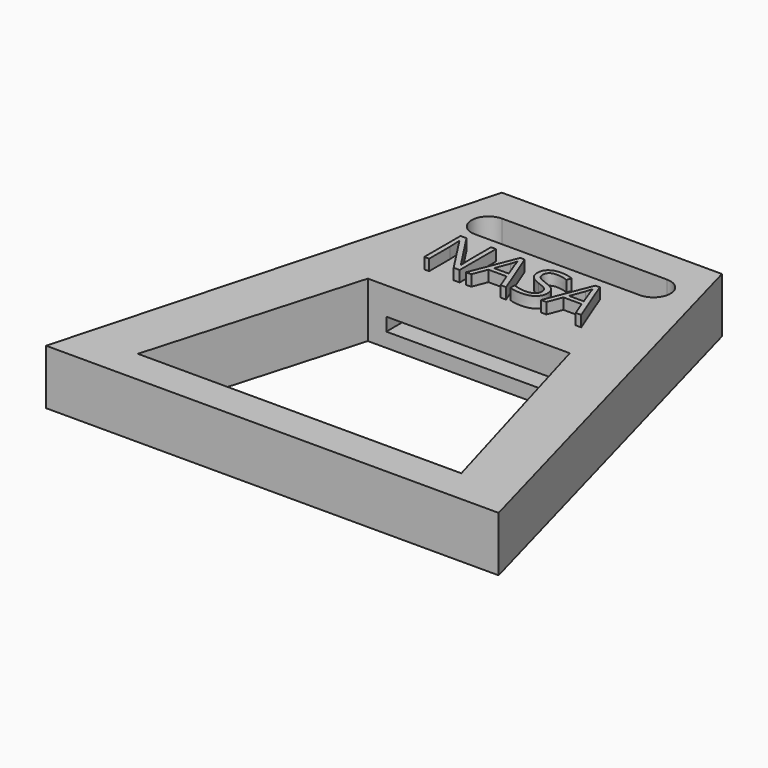
from build123d import *

# Parameters (mm, degrees)
F1_DEPTH     = 6.35
F2_W         = 9.525
F2_H         = 1.52146
F3_DEPTH     = 9.525
F5_TEXT_SIZE = 7.3332446112
F6_DEPTH     = 1.27


# Not quite as in the source:
# - Text() gives the source's letters only with a copy of the font that has no kerning and outlines rounded to 1/6400 em; it was checked with that copy


with BuildPart() as f1:
    # F0 (on Top) → F1 (new body)
    with BuildSketch(Plane.XY):
        with BuildLine():
            Line((0, 25.178215708), (0, 29.1238968258))
            Line((0, 29.1238968258), (-12.7, 29.1238968258))
            Line((-12.7, 29.1238968258), (-26.1181264482, -19.8719589441))
            Line((-26.1181264482, -19.8719589441), (0, -19.8719589441))
            Line((0, -19.8719589441), (0, -15.9369520843))
            Line((0, -15.9369520843), (-18.6689998955, -15.9369520843))
            Line((-18.6689998955, -15.9369520843), (-11.6567891455, 8.4759318174))
            Line((-11.6567891455, 8.4759318174), (0, 8.4759318174))
            Line((0, 8.4759318174), (0, 21.266615708))
            Line((0, 21.266615708), (-9.525, 21.266615708))
            ThreePointArc((-9.525, 21.266615708), (-11.4808, 23.222415708), (-9.525, 25.178215708))
            Line((-9.525, 25.178215708), (0, 25.178215708))
        make_face()
    extrude(amount=F1_DEPTH)

    # F2 (on face) → F3 (cut)
    with BuildSketch(Plane.XZ.offset(-8.4759318174)):
        with Locations((-4.7625, 2.41427)):
            Rectangle(F2_W, F2_H)
    extrude(amount=-F3_DEPTH, mode=Mode.SUBTRACT)

    # F4: F1 across plane


with BuildPart() as f1_1:
    add(f1.part)
    add(f1.part.mirror(Plane.YZ))

    # F5 (on face) → F6 (join)
    with BuildSketch(Plane.XY.offset(6.35)):
        with Locations((-9.525, 13.0554565786)):
            Text('NASA', F5_TEXT_SIZE, font='Open Sans', text_align=(TextAlign.LEFT, TextAlign.BOTTOM))
    extrude(amount=F6_DEPTH)


solid = f1_1.part
